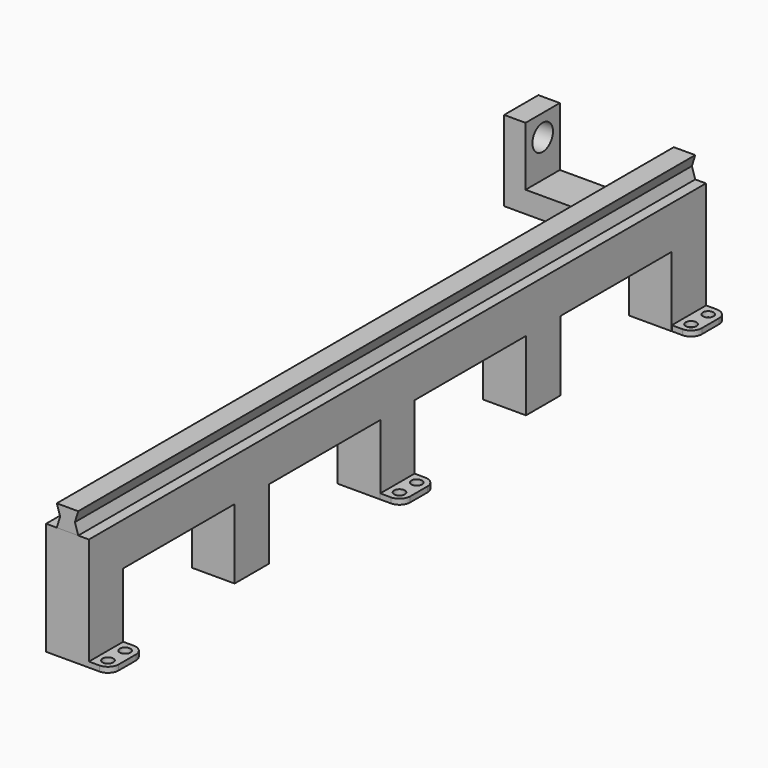
from build123d import *

# Parameters (mm, degrees)
F1_DEPTH  = 50.8
F3_DEPTH  = 914.4
F5_W      = 50.2879026413
F5_H      = 25.4
F6_DEPTH  = 50.8
F8_R      = 6.35
F9_DEPTH  = 6.35
F11_R     = 15.24
F12_DEPTH = 25.4


with BuildPart() as f1:
    # F0 (on Right) → F1 (new body)
    with BuildSketch(Plane.YZ):
        Polygon((914.4, 0), (0, 0), (0, -133.731), (50.8, -133.731), (50.8, -50.8), (215.9, -50.8), (215.9, -133.731), (266.7, -133.731), (266.7, -50.8), (431.8, -50.8), (431.8, -133.731), (482.6, -133.731), (482.6, -50.8), (647.7, -50.8), (647.7, -133.731), (698.5, -133.731), (698.5, -50.8), (863.6, -50.8), (863.6, -133.731), (914.4, -133.731), align=None)
    extrude(amount=F1_DEPTH)

    # F5 (on offset) → F6 (join)
    with BuildSketch(Plane.XZ.offset(-838.2)):
        with Locations((25.1439513206, -38.1)):
            Rectangle(F5_W, F5_H)
        Polygon((0, -50.8), (0, -25.4), (-102.1120973587, -25.4), (-102.1120973587, 44.45), (-127.5120973587, 44.45), (-127.5120973587, -50.8), align=None)
    extrude(amount=-F6_DEPTH)

    # F8 (on offset) → F9 (join)
    with BuildSketch(Plane(origin=(0, 0, -133.731), x_dir=(1, 0, 0), z_dir=(0, 0, -1))):
        with BuildLine():
            Line((63.2052357912, 0), (50.5052357912, 0))
            Line((50.5052357912, 0), (50.5052357912, -50.8))
            Line((50.5052357912, -50.8), (63.2052357912, -50.8))
            ThreePointArc((63.2052357912, -50.8), (72.1854919123, -47.0802561211), (75.9052357912, -38.1))
            Line((75.9052357912, -38.1), (75.9052357912, -12.7))
            ThreePointArc((75.9052357912, -12.7), (72.1854919123, -3.7197438789), (63.2052357912, 0))
        make_face()
        with Locations((63.2052357912, -38.1)):
            Circle(F8_R, mode=Mode.SUBTRACT)
        with Locations((63.2052357912, -12.7)):
            Circle(F8_R, mode=Mode.SUBTRACT)
        with BuildLine():
            Line((63.4224947214, -431.774403286), (50.7224947214, -431.774403286))
            Line((50.7224947214, -431.774403286), (50.7224947214, -482.574403286))
            Line((50.7224947214, -482.574403286), (63.4224947214, -482.574403286))
            ThreePointArc((63.4224947214, -482.574403286), (72.4027508425, -478.854659407), (76.1224947214, -469.874403286))
            Line((76.1224947214, -469.874403286), (76.1224947214, -444.474403286))
            ThreePointArc((76.1224947214, -444.474403286), (72.4027508425, -435.4941471649), (63.4224947214, -431.774403286))
        make_face()
        with Locations((63.4224947214, -469.874403286)):
            Circle(F8_R, mode=Mode.SUBTRACT)
        with Locations((63.4224947214, -444.474403286)):
            Circle(F8_R, mode=Mode.SUBTRACT)
    extrude(amount=-F9_DEPTH)

    # F11 (on face) → F12 (cut)
    with BuildSketch(Plane(origin=(-127.5120973587, 0, 0), x_dir=(0, -1, 0), z_dir=(-1, 0, 0))):
        with Locations((-863.6, 19.05)):
            Circle(F11_R)
    extrude(amount=-F12_DEPTH, mode=Mode.SUBTRACT)


with BuildPart() as f3:
    # F2 (on Front) → F3 (new body)
    with BuildSketch(Plane.XZ):
        Polygon((16.6332703084, 12.7), (12.7, 0), (38.1, 0), (34.1667296916, 12.7), (38.1, 25.4), (12.7, 25.4), align=None)
    extrude(amount=-F3_DEPTH)


with BuildPart() as f9:
    # F8 (on offset) → F9, piece 2 (new body)
    with BuildSketch(Plane(origin=(0, 0, -133.731), x_dir=(1, 0, 0), z_dir=(0, 0, -1))):
        with BuildLine():
            Line((50.8901067078, -863.6876599312), (50.8901067078, -914.4876599312))
            Line((50.8901067078, -914.4876599312), (63.5901067078, -914.4876599312))
            ThreePointArc((63.5901067078, -914.4876599312), (72.5703628289, -910.7679160523), (76.2901067078, -901.7876599312))
            Line((76.2901067078, -901.7876599312), (76.2901067078, -876.3876599312))
            ThreePointArc((76.2901067078, -876.3876599312), (72.5703628289, -867.4074038101), (63.5901067078, -863.6876599312))
            Line((63.5901067078, -863.6876599312), (50.8901067078, -863.6876599312))
        make_face()
        with Locations((63.5901067078, -901.7876599312)):
            Circle(F8_R, mode=Mode.SUBTRACT)
        with Locations((63.5901067078, -876.3876599312)):
            Circle(F8_R, mode=Mode.SUBTRACT)
    extrude(amount=-F9_DEPTH)


solid = Compound([f1.part, f3.part, f9.part])
